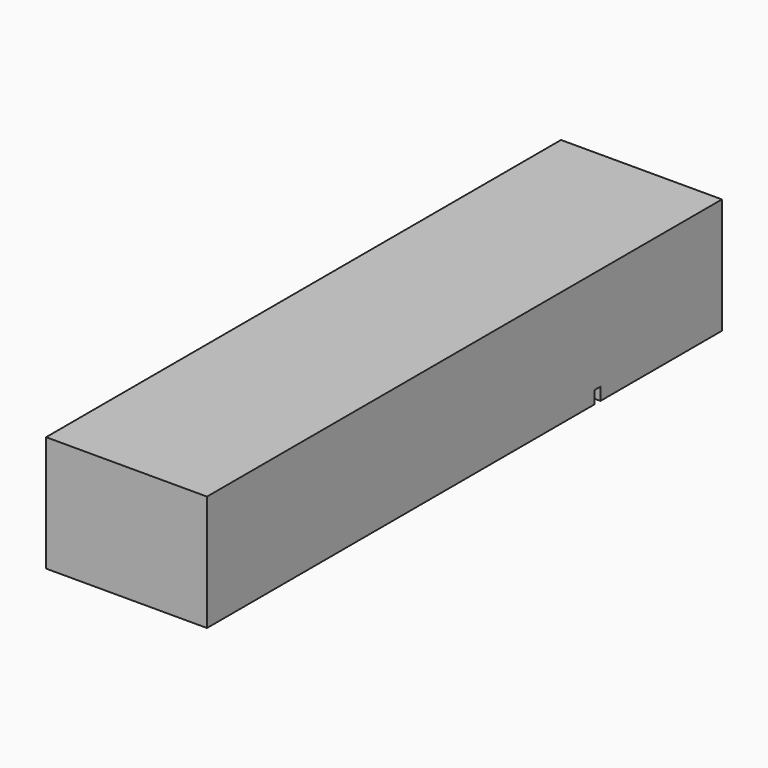
from build123d import *

# Parameters (mm, degrees)
F0_W     = 2
F0_H     = 3.5
F1_DEPTH = 22.25


# Not quite as in the source:
# - a feature of the source that left no trace in its solid (it failed there, or was rolled back) is left out


with BuildPart() as f1:
    # F0 (on Right) → F1 (new body, symmetric)
    with BuildSketch(Plane.YZ):
        Polygon((89, -16), (89, 16), (-89, 16), (-89, -16), (-66, -16), (-66, -12.5), (-64, -12.5), (-64, -16), (45, -16), (45, -12.5), (47, -12.5), (47, -16), align=None)
        with Locations((-65, -14.25)):
            Rectangle(F0_W, F0_H)
    extrude(amount=F1_DEPTH, both=True)


solid = f1.part
